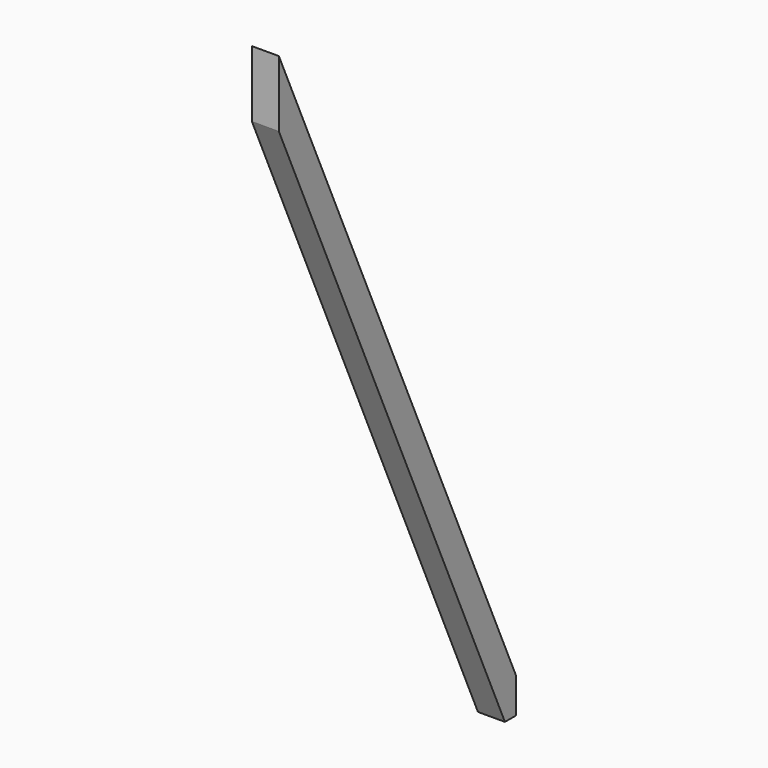
from build123d import *

# Parameters (mm, degrees)
F1_DEPTH = 3.175


# Not quite as in the source:
# - a feature names something its author has since deleted; it is built from what else it names


with BuildPart() as f1:
    # F0 (on Right) → F1 (new body)
    with BuildSketch(Plane.YZ):
        Polygon((1.646842212, 4.1071656714), (-33.278157788, 82.55), (-33.278157788, 74.7439661596), (0, 0), (1.646842212, 0), align=None)
    extrude(amount=F1_DEPTH)


solid = f1.part
